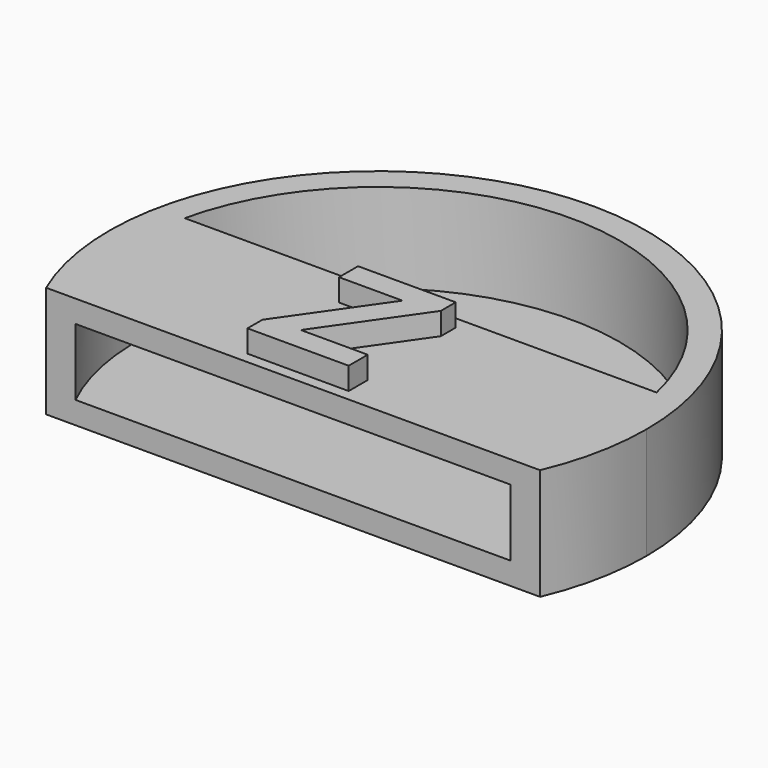
from build123d import *

# Parameters (mm, degrees)
F1_DEPTH     = 5
F0_TEXT_SIZE = 8.5416666667
F2_DEPTH     = 6
F3_DEPTH     = 4
F4_DEPTH     = 1


# Not quite as in the source:
# - a feature names something its author has since deleted; it is built from what else it names
# - Text() gives the source's letters only with a copy of the font that has no kerning and outlines rounded to 1/6400 em; it was checked with that copy


with BuildPart() as f1:
    # F0 (on Top) → F1 (new body)
    with BuildSketch(Plane.XY):
        with BuildLine():
            ThreePointArc((-10.5812333875, 2.4), (-10.7782748651, -1.2455083027), (-9.7549987186, -4.75))
            Line((-9.7549987186, -4.75), (9.7549987186, -4.75))
            ThreePointArc((9.7549987186, -4.75), (10.5727062784, -2.4372898784), (10.85, 0))
            ThreePointArc((10.85, 0), (10.7825989969, 1.2075010861), (10.5812333875, 2.4))
            Line((10.5812333875, 2.4), (0, 2.4))
            Line((0, 2.4), (-10.5812333875, 2.4))
        make_face()
        Polygon((2.0940429688, -3.1822916667), (2.0940429688, -4.25), (-2.4437174479, -4.25), (-2.4437174479, -3.4118489583), (0.48046875, 0.7802408854), (-2.3636393229, 0.7802408854), (-2.3636393229, 1.8479492188), (2.0152994792, 1.8479492188), (2.0152994792, 1.0138020833), (-0.9048828125, -3.1822916667), align=None, mode=Mode.SUBTRACT)
        with BuildLine():
            ThreePointArc((11.0742945599, -4.75), (11.8035534787, -2.4245876508), (12.05, 0))
            ThreePointArc((12.05, 0), (-2.4245876508, 11.8035534787), (-11.0742945599, -4.75))
            Line((-11.0742945599, -4.75), (-9.7549987186, -4.75))
            ThreePointArc((-9.7549987186, -4.75), (-10.7782748651, -1.2455083027), (-10.5812333875, 2.4))
            ThreePointArc((-10.5812333875, 2.4), (0, 10.85), (10.5812333875, 2.4))
            ThreePointArc((10.5812333875, 2.4), (10.7825989969, 1.2075010861), (10.85, 0))
            ThreePointArc((10.85, 0), (10.5727062784, -2.4372898784), (9.7549987186, -4.75))
            Line((9.7549987186, -4.75), (11.0742945599, -4.75))
        make_face()
    extrude(amount=F1_DEPTH)

    # F0 (on Top) → F2 (join)
    with BuildSketch(Plane.XY):
        with Locations((-2.6479166667, -4.25)):
            Text('Z', F0_TEXT_SIZE, font='Open Sans', font_style=FontStyle.BOLD, text_align=(TextAlign.LEFT, TextAlign.BOTTOM))
    extrude(amount=F2_DEPTH)

    # F0 (on Top) → F3 (cut)
    with BuildSketch(Plane.XY):
        with BuildLine():
            ThreePointArc((-10.5812333875, 2.4), (-10.7782748651, -1.2455083027), (-9.7549987186, -4.75))
            Line((-9.7549987186, -4.75), (9.7549987186, -4.75))
            ThreePointArc((9.7549987186, -4.75), (10.5727062784, -2.4372898784), (10.85, 0))
            ThreePointArc((10.85, 0), (10.7825989969, 1.2075010861), (10.5812333875, 2.4))
            Line((10.5812333875, 2.4), (0, 2.4))
            Line((0, 2.4), (-10.5812333875, 2.4))
        make_face()
        Polygon((2.0940429688, -3.1822916667), (2.0940429688, -4.25), (-2.4437174479, -4.25), (-2.4437174479, -3.4118489583), (0.48046875, 0.7802408854), (-2.3636393229, 0.7802408854), (-2.3636393229, 1.8479492188), (2.0152994792, 1.8479492188), (2.0152994792, 1.0138020833), (-0.9048828125, -3.1822916667), align=None, mode=Mode.SUBTRACT)
        with Locations((-2.6479166667, -4.25)):
            Text('Z', F0_TEXT_SIZE, font='Open Sans', font_style=FontStyle.BOLD, text_align=(TextAlign.LEFT, TextAlign.BOTTOM))
    extrude(amount=F3_DEPTH, mode=Mode.SUBTRACT)

    # F0 (on Top) → F4 (join)
    with BuildSketch(Plane.XY):
        with BuildLine():
            ThreePointArc((10.5812333875, 2.4), (0, 10.85), (-10.5812333875, 2.4))
            Line((-10.5812333875, 2.4), (0, 2.4))
            Line((0, 2.4), (10.5812333875, 2.4))
        make_face()
        with BuildLine():
            ThreePointArc((2.35, 4.75), (1.6617009358, 3.0882990642), (0, 2.4))
            ThreePointArc((0, 2.4), (-1.6617009358, 6.4117009358), (2.35, 4.75))
        make_face(mode=Mode.SUBTRACT)
        with BuildLine():
            ThreePointArc((-10.5812333875, 2.4), (-10.7782748651, -1.2455083027), (-9.7549987186, -4.75))
            Line((-9.7549987186, -4.75), (9.7549987186, -4.75))
            ThreePointArc((9.7549987186, -4.75), (10.5727062784, -2.4372898784), (10.85, 0))
            ThreePointArc((10.85, 0), (10.7825989969, 1.2075010861), (10.5812333875, 2.4))
            Line((10.5812333875, 2.4), (0, 2.4))
            Line((0, 2.4), (-10.5812333875, 2.4))
        make_face()
        Polygon((2.0940429688, -3.1822916667), (2.0940429688, -4.25), (-2.4437174479, -4.25), (-2.4437174479, -3.4118489583), (0.48046875, 0.7802408854), (-2.3636393229, 0.7802408854), (-2.3636393229, 1.8479492188), (2.0152994792, 1.8479492188), (2.0152994792, 1.0138020833), (-0.9048828125, -3.1822916667), align=None, mode=Mode.SUBTRACT)
        with Locations((-2.6479166667, -4.25)):
            Text('Z', F0_TEXT_SIZE, font='Open Sans', font_style=FontStyle.BOLD, text_align=(TextAlign.LEFT, TextAlign.BOTTOM))
    extrude(amount=F4_DEPTH)


solid = f1.part
